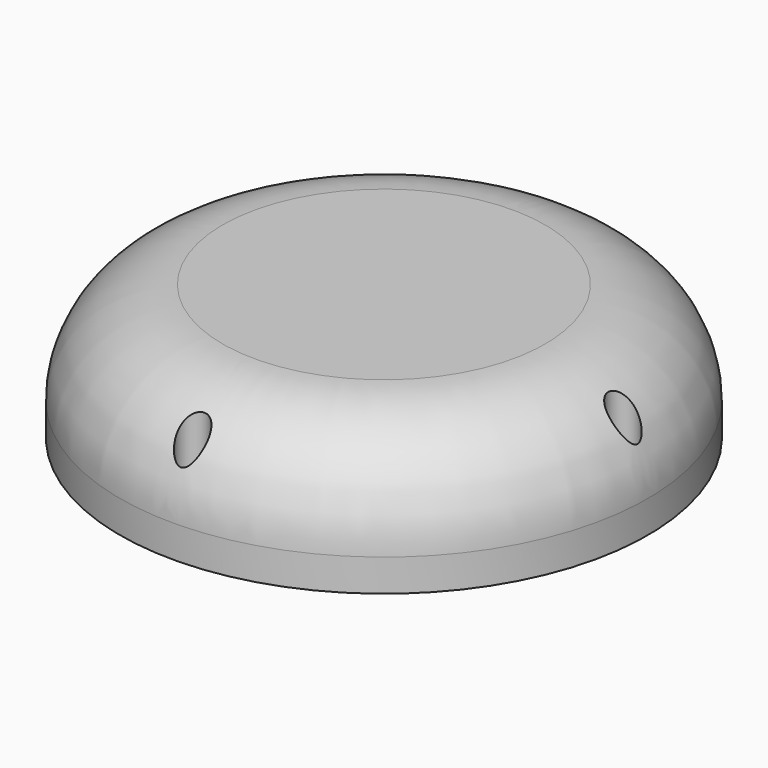
from build123d import *

# Parameters (mm, degrees)
F0_R      = 61
F0_R_2    = 58
F1_DEPTH  = 4
F2_R      = 61
F2_R_2    = 56
F3_DEPTH  = 3
F4_SIZE   = 1.99999
F5_R      = 2.25
F6_DEPTH  = 7
F7_SIZE   = 3
F8_R      = 76
F8_R_2    = 2.25
F9_DEPTH  = 4
F10_W     = 190.4741451144
F10_H     = 3
F10_H_2   = 4
F11_DEPTH = 100
F12_R     = 2.25
F13_DEPTH = 50
F16_DEPTH = 73
F17_R     = 5
F18_DEPTH = 46.7
F20_DEPTH = 400
F21_R     = 73.5
F22_DEPTH = 5
F24_R     = 20


# Not quite as in the source:
# - a fillet or chamfer that OpenCascade refuses, or shapes differently, is made with other operations: its cross-section is extruded or revolved along the edge and cut away or added
# - a fillet or chamfer is up to 0.001 mm smaller than in the source, because OpenCascade refuses the exact size
# - a feature of the source that left no trace in its solid (it failed there, or was rolled back) is left out
# - a feature names something its author has since deleted; it is built from what else it names


with BuildPart() as f1:
    # F0 (on Top) → F1 (new body)
    with BuildSketch(Plane.XY):
        Circle(F0_R)
        Circle(F0_R_2, mode=Mode.SUBTRACT)
    extrude(amount=F1_DEPTH)

    # F2 (on Top) → F3 (join)
    with BuildSketch(Plane.XY):
        Circle(F2_R)
        Circle(F2_R_2, mode=Mode.SUBTRACT)
    extrude(amount=-F3_DEPTH)

    # F4 (size 2 in the source; OpenCascade refuses exactly that, so slightly less here)
    f4_edges = [f1.edges().sort_by_distance(p)[0] for p in [
        (-56, 0, 0),
    ]]
    chamfer(f4_edges, length=F4_SIZE)

    # F5 (on face) → F6 (join)
    with BuildSketch(Plane(origin=(0, 0, -3), x_dir=(1, 0, 0), z_dir=(0, 0, -1))):
        with BuildLine():
            ThreePointArc((-53.9524024645, 46.1781799693), (-46.4524024645, 38.6781799693), (-38.9524024645, 46.1781799693))
            ThreePointArc((-38.9524024645, 46.1781799693), (-41.1922562627, 51.5242871452), (-46.5739656475, 53.6771947308))
            ThreePointArc((-46.5739656475, 53.6771947308), (-51.7985096404, 51.4383261711), (-53.9524024645, 46.1781799693))
        make_face()
        with Locations((-46.4524024645, 46.1781799693)):
            Circle(F5_R, mode=Mode.SUBTRACT)
        with BuildLine():
            ThreePointArc((-46.1781799693, -53.9524024645), (-40.8748791104, -51.7557033234), (-38.6781799693, -46.4524024645))
            ThreePointArc((-38.6781799693, -46.4524024645), (-46.2389635571, -38.9526487781), (-53.6771947308, -46.5739656475))
            ThreePointArc((-53.6771947308, -46.5739656475), (-51.4383261711, -51.7985096404), (-46.1781799693, -53.9524024645))
        make_face()
        with Locations((-46.1781799693, -46.4524024645)):
            Circle(F5_R, mode=Mode.SUBTRACT)
        with BuildLine():
            ThreePointArc((46.5739656475, -53.6771947308), (51.7985096404, -51.4383261711), (53.9524024645, -46.1781799693))
            ThreePointArc((53.9524024645, -46.1781799693), (41.1062952885, -40.9180337676), (46.5739656475, -53.6771947308))
        make_face()
        with Locations((46.4524024645, -46.1781799693)):
            Circle(F5_R, mode=Mode.SUBTRACT)
        with BuildLine():
            ThreePointArc((46.1781799693, 53.9524024645), (40.8748791104, 41.1491016056), (53.6781799693, 46.4524024645))
            ThreePointArc((53.6781799693, 46.4524024645), (53.6779336557, 46.5131860522), (53.6771947308, 46.5739656475))
            ThreePointArc((53.6771947308, 46.5739656475), (51.4383261711, 51.7985096404), (46.1781799693, 53.9524024645))
        make_face()
        with Locations((46.1781799693, 46.4524024645)):
            Circle(F5_R, mode=Mode.SUBTRACT)
        with BuildLine():
            ThreePointArc((-47.1436914684, 38.7101066225), (-51.9947245198, 41.1251940961), (-53.9524024645, 46.1781799693))
            Line((-53.9524024645, 46.1781799693), (-53.9524024645, 28.4629279645))
            ThreePointArc((-53.9524024645, 28.4629279645), (-50.8070489178, 33.7586104611), (-47.1436914684, 38.7101066225))
        make_face()
        with BuildLine():
            Line((-28.4269492748, 53.9713679179), (-46.5739656475, 53.6771947308))
            ThreePointArc((-46.5739656475, 53.6771947308), (-41.4610501615, 51.7760726253), (-38.9885529473, 46.9136732635))
            ThreePointArc((-38.9885529473, 46.9136732635), (-33.8919643636, 50.7181895534), (-28.4269492748, 53.9713679179))
        make_face()
        with BuildLine():
            Line((46.1781799693, 53.9524024645), (28.4629279645, 53.9524024645))
            ThreePointArc((28.4629279645, 53.9524024645), (33.7586104611, 50.8070489178), (38.7101066225, 47.1436914684))
            ThreePointArc((38.7101066225, 47.1436914684), (41.1251940961, 51.9947245198), (46.1781799693, 53.9524024645))
        make_face()
        with BuildLine():
            Line((53.9713679179, 28.4269492748), (53.6771947308, 46.5739656475))
            ThreePointArc((53.6771947308, 46.5739656475), (53.6779336557, 46.5131860522), (53.6781799693, 46.4524024645))
            ThreePointArc((53.6781799693, 46.4524024645), (51.7354364735, 41.4158460866), (46.9136732635, 38.9885529473))
            ThreePointArc((46.9136732635, 38.9885529473), (50.7181895534, 33.8919643636), (53.9713679179, 28.4269492748))
        make_face()
        with BuildLine():
            Line((53.9524024645, -46.1781799693), (53.9524024645, -28.4629279645))
            ThreePointArc((53.9524024645, -28.4629279645), (50.8070489178, -33.7586104611), (47.1436914684, -38.7101066225))
            ThreePointArc((47.1436914684, -38.7101066225), (51.9947245198, -41.1251940961), (53.9524024645, -46.1781799693))
        make_face()
        with BuildLine():
            ThreePointArc((38.9885529473, -46.9136732635), (33.8919643636, -50.7181895534), (28.4269492748, -53.9713679179))
            Line((28.4269492748, -53.9713679179), (46.5739656475, -53.6771947308))
            ThreePointArc((46.5739656475, -53.6771947308), (41.4610501615, -51.7760726253), (38.9885529473, -46.9136732635))
        make_face()
        with BuildLine():
            ThreePointArc((-38.7101066225, -47.1436914684), (-41.1251940961, -51.9947245198), (-46.1781799693, -53.9524024645))
            Line((-46.1781799693, -53.9524024645), (-28.4629279645, -53.9524024645))
            ThreePointArc((-28.4629279645, -53.9524024645), (-33.7586104611, -50.8070489178), (-38.7101066225, -47.1436914684))
        make_face()
        with BuildLine():
            ThreePointArc((-46.9136732635, -38.9885529473), (-50.7181895534, -33.8919643636), (-53.9713679179, -28.4269492748))
            Line((-53.9713679179, -28.4269492748), (-53.6771947308, -46.5739656475))
            ThreePointArc((-53.6771947308, -46.5739656475), (-51.7760726253, -41.4610501615), (-46.9136732635, -38.9885529473))
        make_face()
    extrude(amount=-F6_DEPTH)

    # F7
    f7_edges = [f1.edges().sort_by_distance(p)[0] for p in [
        (43.92818, -46.452402, -3),
        (44.202402, 46.17818, -3),
        (-48.42818, 46.452402, -3),
        (-48.702402, -46.17818, -3),
    ]]
    chamfer(f7_edges, length=F7_SIZE)

    # F8 (on face) → F9 (join)
    with BuildSketch(Plane.XY.offset(4)):
        Circle(F8_R)
        with BuildLine():
            ThreePointArc((53.9524024645, 28.4629279645), (60.9999966103, 0.0203356494), (53.9713679179, -28.4269492748))
            Line((53.9713679179, -28.4269492748), (53.6771947308, -46.5739656475))
            ThreePointArc((53.6771947308, -46.5739656475), (51.4383261711, -51.7985096404), (46.1781799693, -53.9524024644))
            Line((46.1781799693, -53.9524024645), (28.4629279645, -53.9524024645))
            ThreePointArc((28.4629279645, -53.9524024645), (0.0203356494, -60.9999966103), (-28.4269492748, -53.9713679179))
            Line((-28.4269492748, -53.9713679179), (-46.5739656475, -53.6771947308))
            ThreePointArc((-46.5739656475, -53.6771947308), (-51.7985096404, -51.4383261711), (-53.9524024645, -46.1781799693))
            Line((-53.9524024645, -46.1781799693), (-53.9524024645, -28.4629279645))
            ThreePointArc((-53.9524024645, -28.4629279645), (-60.9999966103, -0.0203356494), (-53.9713679179, 28.4269492748))
            Line((-53.9713679179, 28.4269492748), (-53.6771947308, 46.5739656475))
            ThreePointArc((-53.6771947308, 46.5739656475), (-51.4383261711, 51.7985096404), (-46.1781799693, 53.9524024645))
            Line((-46.1781799693, 53.9524024645), (-28.4629279645, 53.9524024645))
            ThreePointArc((-28.4629279645, 53.9524024645), (-0.0203356494, 60.9999966103), (28.4269492748, 53.9713679179))
            Line((28.4269492748, 53.9713679179), (46.5739656475, 53.6771947308))
            ThreePointArc((46.5739656475, 53.6771947308), (51.7985096404, 51.4383261711), (53.9524024645, 46.1781799693))
            Line((53.9524024645, 46.1781799693), (53.9524024645, 28.4629279645))
        make_face(mode=Mode.SUBTRACT)
        with Locations((-46.1781799693, 46.4524024645)):
            Circle(F8_R_2)
    extrude(amount=F9_DEPTH)

    # F10 (on Right) → F11 (cut, symmetric)
    with BuildSketch(Plane.YZ):
        with Locations((-5.4310373962, -1.5)):
            Rectangle(F10_W, F10_H)
        with Locations((-5.4310373962, 2)):
            Rectangle(F10_W, F10_H_2)
    extrude(amount=F11_DEPTH, both=True, mode=Mode.SUBTRACT)

    # F12 (on face) → F13 (join)
    with BuildSketch(Plane(origin=(0, 0, 4), x_dir=(1, 0, 0), z_dir=(0, 0, -1))):
        with BuildLine():
            ThreePointArc((90, 0), (81.5, -8.5), (73, 0))
            ThreePointArc((73, 0), (51.6187950614, -51.6187949919), (9.83e-08, -73))
            ThreePointArc((9.83e-08, -73), (6.0104076749, -75.4895923947), (8.5, -81.5))
            ThreePointArc((8.5, -81.5), (6.0104076196, -87.5104076606), (-5.8e-08, -90))
            ThreePointArc((-5.8e-08, -90), (63.6396102863, -63.6396103273), (90, 0))
        make_face()
        with BuildLine():
            ThreePointArc((9.4e-09, 73), (51.6187950299, 51.6187950233), (73, 0))
            ThreePointArc((73, 0), (81.5, 8.5), (90, 0))
            ThreePointArc((90, 0), (63.6396103068, 63.6396103068), (0, 90))
            ThreePointArc((0, 90), (6.0104076401, 87.5104076401), (8.5, 81.5))
            ThreePointArc((8.5, 81.5), (6.0104076434, 75.4895923632), (9.4e-09, 73))
        make_face()
        with BuildLine():
            ThreePointArc((90, 0), (81.5, 8.5), (73, 0))
            ThreePointArc((73, 0), (81.5, -8.5), (90, 0))
        make_face()
        with Locations((81.5, 0)):
            Circle(F12_R, mode=Mode.SUBTRACT)
        with BuildLine():
            ThreePointArc((-73, 0), (-51.6187950233, 51.6187950299), (9.4e-09, 73))
            ThreePointArc((9.4e-09, 73), (-8.5, 81.4999999953), (0, 90))
            ThreePointArc((0, 90), (-63.6396103153, 63.6396102983), (-90, -2.4e-08))
            ThreePointArc((-90, -2.4e-08), (-81.500000012, 8.5), (-73, 0))
        make_face()
        with BuildLine():
            ThreePointArc((0, 90), (-8.5, 81.4999999953), (9.4e-09, 73))
            ThreePointArc((9.4e-09, 73), (6.0104076434, 75.4895923632), (8.5, 81.5))
            ThreePointArc((8.5, 81.5), (6.0104076401, 87.5104076401), (0, 90))
        make_face()
        with Locations((0, 81.5)):
            Circle(F12_R, mode=Mode.SUBTRACT)
        with BuildLine():
            ThreePointArc((-5.8e-08, -90), (-8.5, -81.4999999219), (9.83e-08, -73))
            ThreePointArc((9.83e-08, -73), (-51.6187949919, -51.6187950614), (-73, 0))
            ThreePointArc((-73, 0), (-81.499999988, -8.5), (-90, -2.4e-08))
            ThreePointArc((-90, -2.4e-08), (-63.6396103188, -63.6396102948), (-5.8e-08, -90))
        make_face()
        with BuildLine():
            ThreePointArc((8.5, -81.5), (6.0104076749, -75.4895923947), (9.83e-08, -73))
            ThreePointArc((9.83e-08, -73), (-8.5, -81.4999999219), (-5.8e-08, -90))
            ThreePointArc((-5.8e-08, -90), (6.0104076196, -87.5104076606), (8.5, -81.5))
        make_face()
        with Locations((0, -81.5)):
            Circle(F12_R, mode=Mode.SUBTRACT)
        with BuildLine():
            ThreePointArc((-90, -2.4e-08), (-81.499999988, -8.5), (-73, 0))
            ThreePointArc((-73, 0), (-81.500000012, 8.5), (-90, -2.4e-08))
        make_face()
        with Locations((-81.5, 0)):
            Circle(F12_R, mode=Mode.SUBTRACT)
    extrude(amount=F13_DEPTH)

    # F12 (on face) → F16 (cut)
    with BuildSketch(Plane(origin=(0, 0, 4), x_dir=(1, 0, 0), z_dir=(0, 0, -1))):
        with Locations((-81.5, 0)):
            Circle(F12_R)
        with Locations((0, -81.5)):
            Circle(F12_R)
        with Locations((81.5, 0)):
            Circle(F12_R)
        with Locations((0, 81.5)):
            Circle(F12_R)
    extrude(amount=F16_DEPTH, mode=Mode.SUBTRACT)

    # F17 (on face) → F18 (cut)
    with BuildSketch(Plane.XY.offset(8)):
        with Locations((0, 81.5)):
            Circle(F17_R)
        with Locations((-81.5, 0)):
            Circle(F17_R)
        with Locations((81.5, 0)):
            Circle(F17_R)
        with Locations((0, -81.5)):
            Circle(F17_R)
    extrude(amount=-F18_DEPTH, mode=Mode.SUBTRACT)

    # F19 (on Right) → F20 (cut, symmetric)
    with BuildSketch(Plane.YZ):
        Polygon((-100.4741415381, 25.2155177295), (-101.8318980932, 0), (102.0258665085, 0), (102.0258665085, 25.2155177295), align=None)
    extrude(amount=F20_DEPTH, both=True, mode=Mode.SUBTRACT)

    # F21 (on face) → F22 (join)
    with BuildSketch(Plane.XY):
        Circle(F21_R)
    extrude(amount=-F22_DEPTH)

    # F23: fillet of radius 35 on 1 edges, made by hand

    # F23_s1 → F23_t2 (revolve, cut)
    with BuildSketch(Plane.XZ):
        with BuildLine():
            ThreePointArc((-55, 0), (-79.7487373415, -10.2512626585), (-90, -35))
            Line((-90, -35), (-90, 0))
            Line((-90, 0), (-55, 0))
        make_face()
    revolve(axis=Axis((0, 0, 0), (0, 0, 1)), mode=Mode.SUBTRACT)

    # F24
    f24_edges = [f1.edges().sort_by_distance(p)[0] for p in [
        (73, 0, -5),
    ]]
    fillet(f24_edges, radius=F24_R)


solid = f1.part
